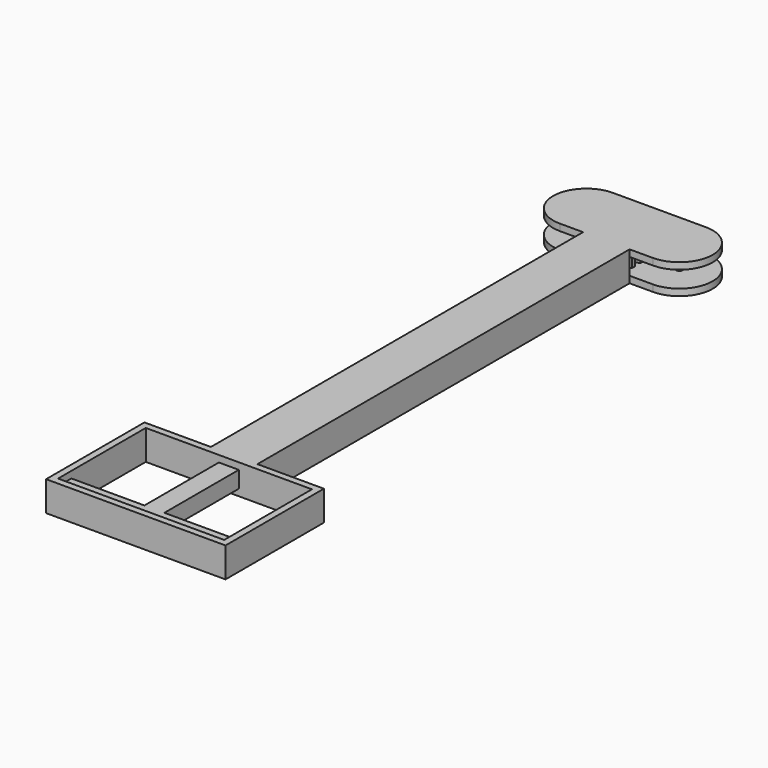
from build123d import *

# Parameters (mm, degrees)
F1_DEPTH      = 5
F3_W          = 50
F3_H          = 5
F4_DEPTH      = 5
F5_W          = 50
F5_H          = 33
F6_DEPTH      = 7
F6_DEPTH_BACK = 2
F9_DEPTH      = 5
F10_W         = 10
F10_H         = 5
F11_DEPTH     = 50
F12_R         = 1
F13_DEPTH     = 5


with BuildPart() as f1:
    # F0 (on Top) → F1 (new body)
    with BuildSketch(Plane.XY):
        Polygon((3, 11.0871235167), (3, 13), (0, 13), (0, -180), (3, -180), (3, -39.0871235167), (3, -36.9128764833), (3, -35.8871235167), (3, -33.7128764833), (3, -32.6871235167), (3, -30.5128764833), (3, -29.4871235167), (3, -27.3128764833), (3, -26.2871235167), (3, -24.1128764833), (3, -23.0871235167), (3, -20.9128764833), (3, -19.8871235167), (3, -17.7128764833), (3, -16.6871235167), (3, -14.5128764833), (3, -13.4871235167), (3, -11.3128764833), (3, -10.2871235167), (3, -8.1128764833), (3, -7.0871235167), (3, -4.9128764833), (3, -3.8871235167), (3, -1.7128764833), (3, -0.6871235167), (3, 1.4871235167), (3, 2.5128764833), (3, 4.6871235167), (3, 5.7128764833), (3, 7.8871235167), (3, 8.9128764833), align=None)
        with BuildLine():
            ThreePointArc((5, 10.5), (4.0421988802, 10.9373096378), (3, 11.0871235167))
            Line((3, 11.0871235167), (3, 8.9128764833))
            ThreePointArc((3, 8.9128764833), (4.0421988802, 9.0626903622), (5, 9.5))
            Line((5, 9.5), (5, 10))
            Line((5, 10), (5, 10.5))
        make_face()
        with BuildLine():
            ThreePointArc((5, 7.3), (4.0421988802, 7.7373096378), (3, 7.8871235167))
            Line((3, 7.8871235167), (3, 5.7128764833))
            ThreePointArc((3, 5.7128764833), (4.0421988802, 5.8626903622), (5, 6.3))
            Line((5, 6.3), (5, 6.8))
            Line((5, 6.8), (5, 7.3))
        make_face()
        with BuildLine():
            Line((3, -36.9128764833), (3, -39.0871235167))
            ThreePointArc((3, -39.0871235167), (4.0421988802, -38.9373096378), (5, -38.5))
            Line((5, -38.5), (5, -38))
            Line((5, -38), (5, -37.5))
            ThreePointArc((5, -37.5), (4.0421988802, -37.0626903622), (3, -36.9128764833))
        make_face()
        with BuildLine():
            ThreePointArc((5, 4.1), (4.0421988802, 4.5373096378), (3, 4.6871235167))
            Line((3, 4.6871235167), (3, 2.5128764833))
            ThreePointArc((3, 2.5128764833), (4.0421988802, 2.6626903622), (5, 3.1))
            Line((5, 3.1), (5, 3.6))
            Line((5, 3.6), (5, 4.1))
        make_face()
        with BuildLine():
            Line((3, -33.7128764833), (3, -35.8871235167))
            ThreePointArc((3, -35.8871235167), (4.0421988802, -35.7373096378), (5, -35.3))
            Line((5, -35.3), (5, -34.8))
            Line((5, -34.8), (5, -34.3))
            ThreePointArc((5, -34.3), (4.0421988802, -33.8626903622), (3, -33.7128764833))
        make_face()
        with BuildLine():
            ThreePointArc((5, 0.9), (4.0421988802, 1.3373096378), (3, 1.4871235167))
            Line((3, 1.4871235167), (3, -0.6871235167))
            ThreePointArc((3, -0.6871235167), (4.0421988802, -0.5373096378), (5, -0.1))
            Line((5, -0.1), (5, 0.4))
            Line((5, 0.4), (5, 0.9))
        make_face()
        with BuildLine():
            Line((3, -30.5128764833), (3, -32.6871235167))
            ThreePointArc((3, -32.6871235167), (4.0421988802, -32.5373096378), (5, -32.1))
            Line((5, -32.1), (5, -31.6))
            Line((5, -31.6), (5, -31.1))
            ThreePointArc((5, -31.1), (4.0421988802, -30.6626903622), (3, -30.5128764833))
        make_face()
        with BuildLine():
            ThreePointArc((5, -2.3), (4.0421988802, -1.8626903622), (3, -1.7128764833))
            Line((3, -1.7128764833), (3, -3.8871235167))
            ThreePointArc((3, -3.8871235167), (4.0421988802, -3.7373096378), (5, -3.3))
            Line((5, -3.3), (5, -2.8))
            Line((5, -2.8), (5, -2.3))
        make_face()
        with BuildLine():
            Line((3, -27.3128764833), (3, -29.4871235167))
            ThreePointArc((3, -29.4871235167), (4.0421988802, -29.3373096378), (5, -28.9))
            Line((5, -28.9), (5, -28.4))
            Line((5, -28.4), (5, -27.9))
            ThreePointArc((5, -27.9), (4.0421988802, -27.4626903622), (3, -27.3128764833))
        make_face()
        with BuildLine():
            ThreePointArc((5, -5.5), (4.0421988802, -5.0626903622), (3, -4.9128764833))
            Line((3, -4.9128764833), (3, -7.0871235167))
            ThreePointArc((3, -7.0871235167), (4.0421988802, -6.9373096378), (5, -6.5))
            Line((5, -6.5), (5, -6))
            Line((5, -6), (5, -5.5))
        make_face()
        with BuildLine():
            Line((3, -24.1128764833), (3, -26.2871235167))
            ThreePointArc((3, -26.2871235167), (4.0421988802, -26.1373096378), (5, -25.7))
            Line((5, -25.7), (5, -25.2))
            Line((5, -25.2), (5, -24.7))
            ThreePointArc((5, -24.7), (4.0421988802, -24.2626903622), (3, -24.1128764833))
        make_face()
        with BuildLine():
            ThreePointArc((5, -8.7), (4.0421988802, -8.2626903622), (3, -8.1128764833))
            Line((3, -8.1128764833), (3, -10.2871235167))
            ThreePointArc((3, -10.2871235167), (4.0421988802, -10.1373096378), (5, -9.7))
            Line((5, -9.7), (5, -9.2))
            Line((5, -9.2), (5, -8.7))
        make_face()
        with BuildLine():
            Line((3, -20.9128764833), (3, -23.0871235167))
            ThreePointArc((3, -23.0871235167), (4.0421988802, -22.9373096378), (5, -22.5))
            Line((5, -22.5), (5, -22))
            Line((5, -22), (5, -21.5))
            ThreePointArc((5, -21.5), (4.0421988802, -21.0626903622), (3, -20.9128764833))
        make_face()
        with BuildLine():
            ThreePointArc((5, -11.9), (4.0421988802, -11.4626903622), (3, -11.3128764833))
            Line((3, -11.3128764833), (3, -13.4871235167))
            ThreePointArc((3, -13.4871235167), (4.0421988802, -13.3373096378), (5, -12.9))
            Line((5, -12.9), (5, -12.4))
            Line((5, -12.4), (5, -11.9))
        make_face()
        with BuildLine():
            Line((3, -17.7128764833), (3, -19.8871235167))
            ThreePointArc((3, -19.8871235167), (4.0421988802, -19.7373096378), (5, -19.3))
            Line((5, -19.3), (5, -18.8))
            Line((5, -18.8), (5, -18.3))
            ThreePointArc((5, -18.3), (4.0421988802, -17.8626903622), (3, -17.7128764833))
        make_face()
        with BuildLine():
            ThreePointArc((5, -15.1), (4.0421988802, -14.6626903622), (3, -14.5128764833))
            Line((3, -14.5128764833), (3, -16.6871235167))
            ThreePointArc((3, -16.6871235167), (4.0421988802, -16.5373096378), (5, -16.1))
            Line((5, -16.1), (5, -15.6))
            Line((5, -15.6), (5, -15.1))
        make_face()
    extrude(amount=F1_DEPTH)

    # F2: F1 across face


with BuildPart() as f1_1:
    add(f1.part)
    add(f1.part.mirror(Plane(origin=(0, -83.5, 2.5), x_dir=(0, -1, 0), z_dir=(-1, 0, 0))))

    # F3 (on face) → F4 (join)
    with BuildSketch(Plane.XZ.offset(180)):
        with Locations((0, 2.5)):
            Rectangle(F3_W, F3_H)
    extrude(amount=F4_DEPTH)


with BuildPart() as f6:
    # F5 (on Top) → F6 (new body, two sides)
    with BuildSketch(Plane.XY) as f6_sk:
        with BuildLine():
            ThreePointArc((14, -10), (21.0710678119, -7.0710678119), (24, 0))
            ThreePointArc((24, 0), (21.0710678119, 7.0710678119), (14, 10))
            ThreePointArc((14, 10), (4, 0), (14, -10))
        make_face()
        with BuildLine():
            ThreePointArc((14, -10), (4, 0), (14, 10))
            Line((14, 10), (0, 10))
            Line((0, 10), (-14, 10))
            ThreePointArc((-14, 10), (-6.9289321881, 7.0710678119), (-4, 0))
            ThreePointArc((-4, 0), (-6.9289321881, -7.0710678119), (-14, -10))
            Line((-14, -10), (-7, -10))
            Line((-7, -10), (-7, -150))
            Line((-7, -150), (-27, -150))
            Line((-27, -150), (-27, -187))
            Line((-27, -187), (0, -187))
            Line((0, -187), (27, -187))
            Line((27, -187), (27, -150))
            Line((27, -150), (7, -150))
            Line((7, -150), (7, -10))
            Line((7, -10), (14, -10))
        make_face()
        with Locations((0, -168.5)):
            Rectangle(F5_W, F5_H, mode=Mode.SUBTRACT)
        with BuildLine():
            ThreePointArc((-4, 0), (-6.9289321881, 7.0710678119), (-14, 10))
            ThreePointArc((-14, 10), (-24, 0), (-14, -10))
            ThreePointArc((-14, -10), (-6.9289321881, -7.0710678119), (-4, 0))
        make_face()
    extrude(amount=F6_DEPTH)
    extrude(f6_sk.sketch, amount=-F6_DEPTH_BACK)

    # F7: cut F1
    add(f1_1.part, mode=Mode.SUBTRACT)

    # F8 (on Top) → F9 (cut)
    with BuildSketch(Plane.XY):
        with BuildLine():
            ThreePointArc((-14, 10), (-24, 0), (-14, -10))
            Line((-14, -10), (14, -10))
            ThreePointArc((14, -10), (24, 0), (14, 10))
            Line((14, 10), (-14, 10))
        make_face()
    extrude(amount=F9_DEPTH, mode=Mode.SUBTRACT)

    # F10 (on face) → F11 (cut)
    with BuildSketch(Plane(origin=(0, -10, 0), x_dir=(-1, 0, 0), z_dir=(0, 1, 0))):
        with Locations((0, 2.5)):
            Rectangle(F10_W, F10_H)
    extrude(amount=-F11_DEPTH, mode=Mode.SUBTRACT)

    # F12 (on Top) → F13 (join, through all)
    with BuildSketch(Plane.XY):
        with Locations((-14, 0)):
            Circle(F12_R)
        with Locations((14, 0)):
            Circle(F12_R)
    extrude(amount=F13_DEPTH)


solid = Compound([f1_1.part, f6.part])
